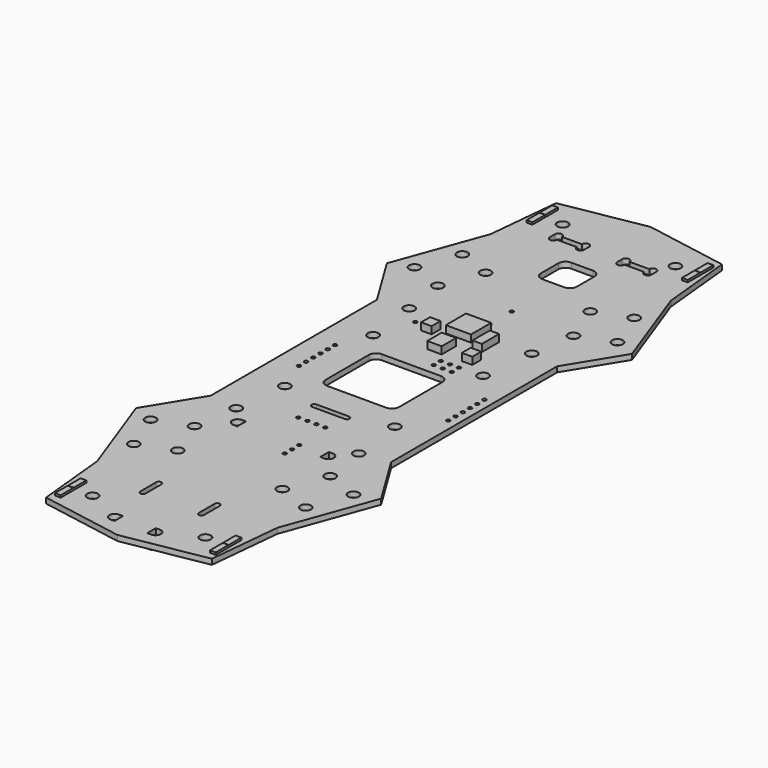
from build123d import *

# Parameters (mm, degrees)
F1_DEPTH  = 1.5
F2_W      = 10
F2_H      = 10
F2_W_2    = 20.4
F2_H_2    = 19
F2_R      = 0.5
F2_R_2    = 1.5
F2_W_3    = 5.5
F2_H_3    = 1.75
F3_DEPTH  = 1.5
F4_W      = 1.6
F4_H      = 4.4
F5_DEPTH  = 0.6
F4_W_2    = 4.4
F4_H_2    = 1.6
F6_R      = 2
F7_W      = 1.6
F7_H      = 4.4
F8_DEPTH  = 0.6
F9_W      = 7
F9_H      = 7
F10_DEPTH = 2
F9_W_2    = 2.6
F9_H_2    = 6
F9_W_3    = 2.9
F9_H_3    = 3.1
F9_W_4    = 4
F9_H_4    = 5


# Not quite as in the source:
# - a feature names something its author has since deleted; it is built from what else it names


with BuildPart() as f1:
    # F0 (on Top) → F1 (new body)
    with BuildSketch(Plane.XY):
        Polygon((-25, 121.3), (-25, 92.5), (-25, 63.7), (-34, 49), (-25, 24.3), (-23, 4.0555205563), (0, 0), (23, 4.0555205563), (25, 24.3), (34, 49), (25, 63.7), (25, 92.5), (25, 121.3), (34, 136), (25, 160.7), (23, 180.9444794437), (0, 185), (-23, 180.9444794437), (-25, 160.7), (-34, 136), align=None)
    extrude(amount=F1_DEPTH)

    # F2 (on face) → F3 (cut, through all)
    with BuildSketch(Plane.XY):
        with Locations((0, 156.2)):
            Rectangle(F2_W, F2_H)
        with Locations((0, 92.5)):
            Rectangle(F2_W_2, F2_H_2)
        with BuildLine():
            ThreePointArc((-8.85, 19.05), (-8.1, 18.3), (-7.35, 19.05))
            Line((-7.35, 19.05), (-7.35, 24.55))
            ThreePointArc((-7.35, 24.55), (-8.1, 25.3), (-8.85, 24.55))
            Line((-8.85, 24.55), (-8.85, 19.05))
        make_face()
        with BuildLine():
            ThreePointArc((-4.5, 74.75), (-5.25, 74), (-4.5, 73.25))
            Line((-4.5, 73.25), (4.5, 73.25))
            ThreePointArc((4.5, 73.25), (5.25, 74), (4.5, 74.75))
            Line((4.5, 74.75), (-4.5, 74.75))
        make_face()
        with BuildLine():
            Line((-11.5, 59), (-12.6, 59))
            ThreePointArc((-12.6, 59), (-14.1, 57.5), (-12.6, 56))
            Line((-12.6, 56), (-11.5, 56))
            Line((-11.5, 56), (-11.5, 59))
        make_face()
        with BuildLine():
            ThreePointArc((12.6, 56), (14.1, 57.5), (12.6, 59))
            Line((12.6, 59), (11.5, 59))
            Line((11.5, 59), (11.5, 56))
            Line((11.5, 56), (12.6, 56))
        make_face()
        with BuildLine():
            Line((-4.55, 7.7), (-5.65, 7.7))
            ThreePointArc((-5.65, 7.7), (-7.15, 6.2), (-5.65, 4.7))
            Line((-5.65, 4.7), (-4.55, 4.7))
            Line((-4.55, 4.7), (-4.55, 7.7))
        make_face()
        with BuildLine():
            Line((4.55, 7.7), (4.55, 4.7))
            Line((4.55, 4.7), (5.65, 4.7))
            ThreePointArc((5.65, 4.7), (7.15, 6.2), (5.65, 7.7))
            Line((5.65, 7.7), (4.55, 7.7))
        make_face()
        with Locations((4.5, 57.5)):
            Circle(F2_R)
        with Locations((4.5, 55)):
            Circle(F2_R)
        with Locations((4.5, 52.5)):
            Circle(F2_R)
        with Locations((-18.8, 99)):
            Circle(F2_R)
        with Locations((-18.8, 96.5)):
            Circle(F2_R)
        with Locations((-18.8, 94)):
            Circle(F2_R)
        with Locations((-18.8, 91.5)):
            Circle(F2_R)
        with Locations((-18.8, 89)):
            Circle(F2_R)
        with Locations((-18.8, 86.5)):
            Circle(F2_R)
        with Locations((22.5, 99.2)):
            Circle(F2_R)
        with Locations((22.5, 96.7)):
            Circle(F2_R)
        with Locations((22.5, 94.2)):
            Circle(F2_R)
        with Locations((22.5, 91.7)):
            Circle(F2_R)
        with Locations((22.5, 89.2)):
            Circle(F2_R)
        with Locations((22.5, 86.7)):
            Circle(F2_R)
        with Locations((3.8, 107.5)):
            Circle(F2_R)
        with Locations((3.8, 105)):
            Circle(F2_R)
        with Locations((6.3, 107.5)):
            Circle(F2_R)
        with Locations((6.3, 105)):
            Circle(F2_R)
        with Locations((8.8, 107.5)):
            Circle(F2_R)
        with Locations((8.8, 105)):
            Circle(F2_R)
        with Locations((-12, 118.3)):
            Circle(F2_R)
        with Locations((-9.5, 118.3)):
            Circle(F2_R)
        with Locations((1.2492573587, 135.1845413446)):
            Circle(F2_R)
        with Locations((1.2492573587, 127.5478899479)):
            Circle(F2_R)
        with Locations((-3.75, 67.5)):
            Circle(F2_R)
        with Locations((-1.25, 67.5)):
            Circle(F2_R)
        with Locations((1.25, 67.5)):
            Circle(F2_R)
        with Locations((3.75, 67.5)):
            Circle(F2_R)
        with Locations((-15.65, 11)):
            Circle(F2_R_2)
        with Locations((15.65, 11)):
            Circle(F2_R_2)
        with BuildLine():
            Line((7.35, 24.55), (7.35, 19.05))
            ThreePointArc((7.35, 19.05), (8.1, 18.3), (8.85, 19.05))
            Line((8.85, 19.05), (8.85, 24.55))
            ThreePointArc((8.85, 24.55), (8.1, 25.3), (7.35, 24.55))
        make_face()
        with Locations((-23.85, 35.53)):
            Circle(F2_R_2)
        with Locations((-28.15, 46.7331245642)):
            Circle(F2_R_2)
        with Locations((-14.5140628632, 39.1133333333)):
            Circle(F2_R_2)
        with Locations((-18.8140628632, 50.3164578975)):
            Circle(F2_R_2)
        with Locations((23.85, 35.53)):
            Circle(F2_R_2)
        with Locations((14.5140628632, 39.1133333333)):
            Circle(F2_R_2)
        with Locations((18.8140628632, 50.3164578975)):
            Circle(F2_R_2)
        with Locations((28.15, 46.7331245642)):
            Circle(F2_R_2)
        with Locations((-17, 62.5)):
            Circle(F2_R_2)
        with Locations((-15.25, 77.2)):
            Circle(F2_R_2)
        with Locations((17, 62.5)):
            Circle(F2_R_2)
        with Locations((15.25, 77.2)):
            Circle(F2_R_2)
        with Locations((-15.25, 107.8)):
            Circle(F2_R_2)
        with Locations((15.25, 107.8)):
            Circle(F2_R_2)
        with Locations((-17, 122.5)):
            Circle(F2_R_2)
        with Locations((17, 122.5)):
            Circle(F2_R_2)
        with Locations((-28.15, 138.2668754358)):
            Circle(F2_R_2)
        with Locations((-18.8140628632, 134.6835421025)):
            Circle(F2_R_2)
        with Locations((-14.5140628632, 145.8866666667)):
            Circle(F2_R_2)
        with Locations((-23.85, 149.47)):
            Circle(F2_R_2)
        with Locations((18.8140628632, 134.6835421025)):
            Circle(F2_R_2)
        with Locations((28.15, 138.2668754358)):
            Circle(F2_R_2)
        with Locations((14.5140628632, 145.8866666667)):
            Circle(F2_R_2)
        with Locations((23.85, 149.47)):
            Circle(F2_R_2)
        with Locations((-15.65, 174)):
            Circle(F2_R_2)
        with Locations((15.65, 174)):
            Circle(F2_R_2)
        with BuildLine():
            ThreePointArc((-12.1, 169.375), (-13.1, 170.375), (-14.1, 169.375))
            Line((-14.1, 169.375), (-14.1, 167.625))
            ThreePointArc((-14.1, 167.625), (-13.1, 166.625), (-12.1, 167.625))
            Line((-12.1, 167.625), (-12.1, 169.375))
        make_face()
        with Locations((-9.35, 168.5)):
            Rectangle(F2_W_3, F2_H_3)
        with BuildLine():
            ThreePointArc((-4.6, 169.375), (-5.6, 170.375), (-6.6, 169.375))
            Line((-6.6, 169.375), (-6.6, 167.625))
            ThreePointArc((-6.6, 167.625), (-5.6, 166.625), (-4.6, 167.625))
            Line((-4.6, 167.625), (-4.6, 169.375))
        make_face()
        with BuildLine():
            Line((12.1, 169.375), (12.1, 167.625))
            ThreePointArc((12.1, 167.625), (13.1, 166.625), (14.1, 167.625))
            Line((14.1, 167.625), (14.1, 169.375))
            ThreePointArc((14.1, 169.375), (13.1, 170.375), (12.1, 169.375))
        make_face()
        with Locations((9.35, 168.5)):
            Rectangle(F2_W_3, F2_H_3)
        with BuildLine():
            ThreePointArc((4.6, 167.625), (5.6, 166.625), (6.6, 167.625))
            Line((6.6, 167.625), (6.6, 169.375))
            ThreePointArc((6.6, 169.375), (5.6, 170.375), (4.6, 169.375))
            Line((4.6, 169.375), (4.6, 167.625))
        make_face()
    extrude(amount=F3_DEPTH, mode=Mode.SUBTRACT)

    # F6
    f6_edges = [f1.edges().sort_by_distance(p)[0] for p in [
        (-10.2, 102, 0.75),
        (10.2, 83, 0.75),
        (-10.2, 83, 0.75),
        (10.2, 102, 0.75),
        (-5, 151.2, 0.75),
        (5, 161.2, 0.75),
        (-5, 161.2, 0.75),
        (5, 151.2, 0.75),
    ]]
    fillet(f6_edges, radius=F6_R)

    # F7 (on face) → F8 (join)
    with BuildSketch(Plane.XY.offset(1.5)):
        with Locations((-21.4829035103, 176.5049248934)):
            Rectangle(F7_W, F7_H)
        with Locations((-21.4829035103, 172.0049248934)):
            Rectangle(F7_W, F7_H)
        with Locations((21.7054244131, 176.3981729746)):
            Rectangle(F7_W, F7_H)
        with Locations((21.7054244131, 171.8981729746)):
            Rectangle(F7_W, F7_H)
        with Locations((21.724851802, 12.6964002848)):
            Rectangle(F7_W, F7_H)
        with Locations((21.724851802, 8.1964002848)):
            Rectangle(F7_W, F7_H)
        with Locations((-21.2847534567, 12.6845447421)):
            Rectangle(F7_W, F7_H)
        with Locations((-21.2847534567, 8.1845447421)):
            Rectangle(F7_W, F7_H)
    extrude(amount=F8_DEPTH)


with BuildPart() as f5:
    # F4 (on face) → F5 (new body)
    with BuildSketch(Plane.XY):
        with Locations((-21.3048513979, 8.0831497908)):
            Rectangle(F4_W, F4_H)
    extrude(amount=-F5_DEPTH)


with BuildPart() as f5b:
    # F4 (on face) → F5, piece 2 (new body)
    with BuildSketch(Plane.XY):
        with Locations((-21.3048513979, 12.8869479522)):
            Rectangle(F4_W, F4_H)
    extrude(amount=-F5_DEPTH)


with BuildPart() as f5c:
    # F4 (on face) → F5, piece 3 (new body)
    with BuildSketch(Plane.XY):
        with Locations((-22.3962776363, 18.7585987151)):
            Rectangle(F4_W, F4_H)
    extrude(amount=-F5_DEPTH)


with BuildPart() as f5d:
    # F4 (on face) → F5, piece 4 (new body)
    with BuildSketch(Plane.XY):
        with Locations((-22.3962776363, 23.5035344958)):
            Rectangle(F4_W, F4_H)
    extrude(amount=-F5_DEPTH)


with BuildPart() as f5e:
    # F4 (on face) → F5, piece 5 (new body)
    with BuildSketch(Plane.XY):
        with Locations((10.2968551219, 7.3306034319)):
            Rectangle(F4_W, F4_H)
    extrude(amount=-F5_DEPTH)


with BuildPart() as f5f:
    # F4 (on face) → F5, piece 6 (new body)
    with BuildSketch(Plane.XY):
        with Locations((-1.2623253278, 7.2313835844)):
            Rectangle(F4_W, F4_H)
    extrude(amount=-F5_DEPTH)


with BuildPart() as f5g:
    # F4 (on face) → F5, piece 7 (new body)
    with BuildSketch(Plane.XY):
        with Locations((-9.0015185997, 6.6924788989)):
            Rectangle(F4_W, F4_H)
    extrude(amount=-F5_DEPTH)


with BuildPart() as f5h:
    # F4 (on face) → F5, piece 8 (new body)
    with BuildSketch(Plane.XY):
        with Locations((-9.0015185997, 11.2994210795)):
            Rectangle(F4_W, F4_H)
    extrude(amount=-F5_DEPTH)


with BuildPart() as f5i:
    # F4 (on face) → F5, piece 9 (new body)
    with BuildSketch(Plane.XY):
        with Locations((21.285880357, 8.0831497908)):
            Rectangle(F4_W, F4_H)
    extrude(amount=-F5_DEPTH)


with BuildPart() as f5j:
    # F4 (on face) → F5, piece 10 (new body)
    with BuildSketch(Plane.XY):
        with Locations((21.285880357, 12.7789328049)):
            Rectangle(F4_W, F4_H)
    extrude(amount=-F5_DEPTH)


with BuildPart() as f5k:
    # F4 (on face) → F5, piece 11 (new body)
    with BuildSketch(Plane.XY):
        with Locations((22.55384624, 18.7585987151)):
            Rectangle(F4_W, F4_H)
    extrude(amount=-F5_DEPTH)


with BuildPart() as f5l:
    # F4 (on face) → F5, piece 12 (new body)
    with BuildSketch(Plane.XY):
        with Locations((22.55384624, 23.4214384109)):
            Rectangle(F4_W, F4_H)
    extrude(amount=-F5_DEPTH)


with BuildPart() as f5m:
    # F4 (on face) → F5, piece 13 (new body)
    with BuildSketch(Plane.XY):
        with Locations((-14.4586423412, 4.998923745)):
            Rectangle(F4_W_2, F4_H_2)
    extrude(amount=-F5_DEPTH)


with BuildPart() as f5n:
    # F4 (on face) → F5, piece 14 (new body)
    with BuildSketch(Plane.XY):
        with Locations((-4.6358196996, 2.9649045318)):
            Rectangle(F4_W_2, F4_H_2)
    extrude(amount=-F5_DEPTH)


with BuildPart() as f5o:
    # F4 (on face) → F5, piece 15 (new body)
    with BuildSketch(Plane.XY):
        with Locations((5.4846638814, 2.9649045318)):
            Rectangle(F4_W_2, F4_H_2)
    extrude(amount=-F5_DEPTH)


with BuildPart() as f5p:
    # F4 (on face) → F5, piece 16 (new body)
    with BuildSketch(Plane.XY):
        with Locations((14.8113835603, 4.8997029662)):
            Rectangle(F4_W_2, F4_H_2)
    extrude(amount=-F5_DEPTH)


with BuildPart() as f5q:
    # F4 (on face) → F5, piece 17 (new body)
    with BuildSketch(Plane.XY):
        with Locations((21.6013076335, 176.4485463619)):
            Rectangle(F4_W, F4_H)
    extrude(amount=-F5_DEPTH)


with BuildPart() as f5r:
    # F4 (on face) → F5, piece 18 (new body)
    with BuildSketch(Plane.XY):
        with Locations((21.6013076335, 172.0292344809)):
            Rectangle(F4_W, F4_H)
    extrude(amount=-F5_DEPTH)


with BuildPart() as f5s:
    # F4 (on face) → F5, piece 19 (new body)
    with BuildSketch(Plane.XY):
        with Locations((20.1874165416, 166.5761098385)):
            Rectangle(F4_W, F4_H)
    extrude(amount=-F5_DEPTH)


with BuildPart() as f5t:
    # F4 (on face) → F5, piece 20 (new body)
    with BuildSketch(Plane.XY):
        with Locations((23.0151987255, 164.3188521385)):
            Rectangle(F4_W, F4_H)
    extrude(amount=-F5_DEPTH)


with BuildPart() as f5u:
    # F4 (on face) → F5, piece 21 (new body)
    with BuildSketch(Plane.XY):
        with Locations((11.8032912344, 178.5073652983)):
            Rectangle(F4_W, F4_H)
    extrude(amount=-F5_DEPTH)


with BuildPart() as f5v:
    # F4 (on face) → F5, piece 22 (new body)
    with BuildSketch(Plane.XY):
        with Locations((4.4755861163, 177.1282404661)):
            Rectangle(F4_W, F4_H)
    extrude(amount=-F5_DEPTH)


with BuildPart() as f5w:
    # F4 (on face) → F5, piece 23 (new body)
    with BuildSketch(Plane.XY):
        with Locations((-8.2919630602, 177.1678850174)):
            Rectangle(F4_W, F4_H)
    extrude(amount=-F5_DEPTH)


with BuildPart() as f5x:
    # F4 (on face) → F5, piece 24 (new body)
    with BuildSketch(Plane.XY):
        with Locations((-5.9101558122, 177.1678850174)):
            Rectangle(F4_W, F4_H)
    extrude(amount=-F5_DEPTH)


with BuildPart() as f5y:
    # F4 (on face) → F5, piece 25 (new body)
    with BuildSketch(Plane.XY):
        with Locations((-21.8361826062, 176.7960563421)):
            Rectangle(F4_W, F4_H)
    extrude(amount=-F5_DEPTH)


with BuildPart() as f5z:
    # F4 (on face) → F5, piece 26 (new body)
    with BuildSketch(Plane.XY):
        with Locations((-21.8361826062, 171.9805821896)):
            Rectangle(F4_W, F4_H)
    extrude(amount=-F5_DEPTH)


with BuildPart() as f5ba:
    # F4 (on face) → F5, piece 27 (new body)
    with BuildSketch(Plane.XY):
        with Locations((-18.6108877331, 167.1466305971)):
            Rectangle(F4_W, F4_H)
    extrude(amount=-F5_DEPTH)


with BuildPart() as f5bb:
    # F4 (on face) → F5, piece 28 (new body)
    with BuildSketch(Plane.XY):
        with Locations((-22.9064566463, 164.5385101557)):
            Rectangle(F4_W, F4_H)
    extrude(amount=-F5_DEPTH)


with BuildPart() as f5bc:
    # F4 (on face) → F5, piece 29 (new body)
    with BuildSketch(Plane.XY):
        with Locations((16.2434051365, 179.8716560125)):
            Rectangle(F4_W_2, F4_H_2)
    extrude(amount=-F5_DEPTH)


with BuildPart() as f5bd:
    # F4 (on face) → F5, piece 30 (new body)
    with BuildSketch(Plane.XY):
        with Locations((5.5740922309, 181.5832033873)):
            Rectangle(F4_W_2, F4_H_2)
    extrude(amount=-F5_DEPTH)


with BuildPart() as f5be:
    # F4 (on face) → F5, piece 31 (new body)
    with BuildSketch(Plane.XY):
        with Locations((-4.1647194885, 181.5009117126)):
            Rectangle(F4_W_2, F4_H_2)
    extrude(amount=-F5_DEPTH)


with BuildPart() as f5bf:
    # F4 (on face) → F5, piece 32 (new body)
    with BuildSketch(Plane.XY):
        with Locations((-17.5690730482, 179.5491799831)):
            Rectangle(F4_W_2, F4_H_2)
    extrude(amount=-F5_DEPTH)


with BuildPart() as f10:
    # F9 (on face) → F10 (new body)
    with BuildSketch(Plane.XY.offset(1.5)):
        with Locations((0, 121.8)):
            Rectangle(F9_W, F9_H)
    extrude(amount=F10_DEPTH)


with BuildPart() as f10b:
    # F9 (on face) → F10, piece 2 (new body)
    with BuildSketch(Plane.XY.offset(1.5)):
        with Locations((6.8, 119.3)):
            Rectangle(F9_W_2, F9_H_2)
    extrude(amount=F10_DEPTH)


with BuildPart() as f10c:
    # F9 (on face) → F10, piece 3 (new body)
    with BuildSketch(Plane.XY.offset(1.5)):
        with Locations((8.8, 111.85)):
            Rectangle(F9_W_3, F9_H_3)
    extrude(amount=F10_DEPTH)


with BuildPart() as f10d:
    # F9 (on face) → F10, piece 4 (new body)
    with BuildSketch(Plane.XY.offset(1.5)):
        with Locations((0, 112.5)):
            Rectangle(F9_W_4, F9_H_4)
    extrude(amount=F10_DEPTH)


with BuildPart() as f10e:
    # F9 (on face) → F10, piece 5 (new body)
    with BuildSketch(Plane.XY.offset(1.5)):
        with Locations((-7.05, 117.55)):
            Rectangle(F9_W_3, F9_H_3)
    extrude(amount=F10_DEPTH)


solid = Compound([f1.part, f5.part, f5b.part, f5c.part, f5d.part, f5e.part, f5f.part, f5g.part, f5h.part, f5i.part, f5j.part, f5k.part, f5l.part, f5m.part, f5n.part, f5o.part, f5p.part, f5q.part, f5r.part, f5s.part, f5t.part, f5u.part, f5v.part, f5w.part, f5x.part, f5y.part, f5z.part, f5ba.part, f5bb.part, f5bc.part, f5bd.part, f5be.part, f5bf.part, f10.part, f10b.part, f10c.part, f10d.part, f10e.part])
